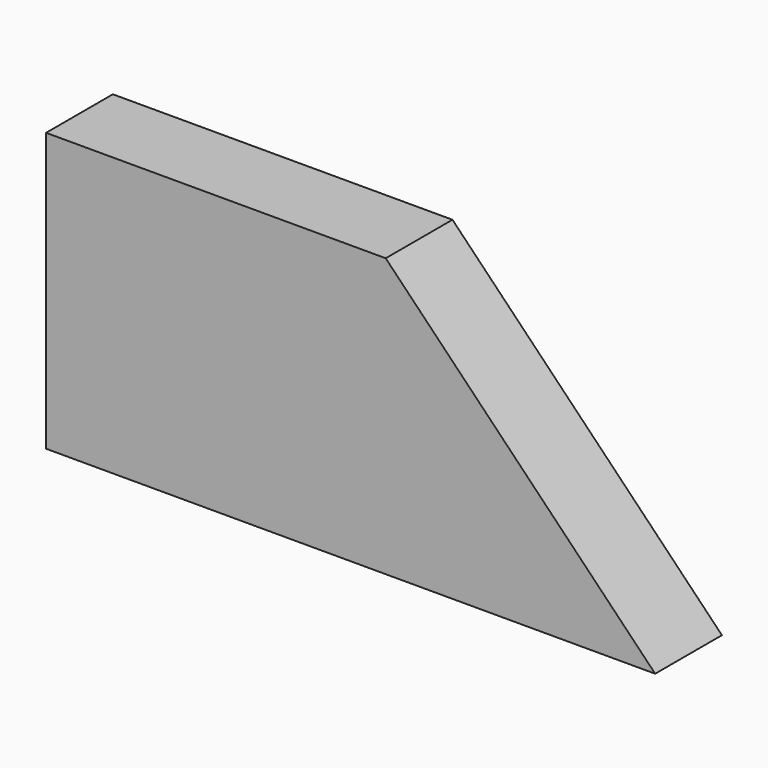
from build123d import *

# Parameters (mm, degrees)
F1_DEPTH = 19.05


# Not quite as in the source:
# - a feature names something its author has since deleted; it is built from what else it names


with BuildPart() as f1:
    # F0 (on Front) → F1 (new body)
    with BuildSketch(Plane.XZ):
        Polygon((77.535532, 63.5), (0, 63.5), (0, 0), (139.0511571057, 0), align=None)
    extrude(amount=F1_DEPTH)


solid = f1.part
